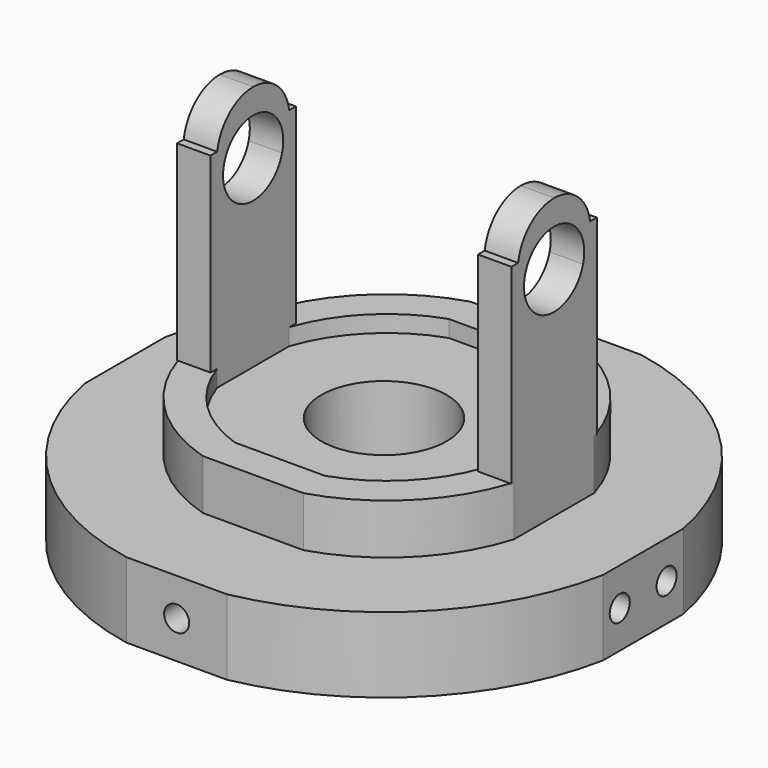
from build123d import *

# Parameters (mm, degrees)
F1_DEPTH  = 6
F2_T      = -4
F3_DEPTH  = 25.4
F4_W      = 10.761987894
F4_H      = 6
F4_H_2    = 27.5
F5_DEPTH  = 4
F6_W      = 10.761987894
F6_H      = 6
F6_H_2    = 27.5
F7_DEPTH  = 4
F9_DEPTH  = 50
F10_DEPTH = 50
F11_DEPTH = 50
F12_DEPTH = 1
F13_DEPTH = 1
F14_DEPTH = 1
F15_DEPTH = 1
F18_DEPTH = 4
F20_DEPTH = 9
F21_R     = 1.5
F22_DEPTH = 7
F23_R     = 1.5
F24_DEPTH = 7
F25_R     = 1.5
F26_DEPTH = 7
F27_R     = 1.5
F28_DEPTH = 7
F29_R     = 7.5
F30_DEPTH = 25.4


with BuildPart() as f1:
    # F0 (on Top) → F1 (new body)
    with BuildSketch(Plane.XY):
        with BuildLine():
            Line((6.0000014261, 20.4372135154), (1.4261e-06, 20.4372135154))
            Line((1.4261e-06, 20.4372135154), (-5.9999985739, 20.4372135154))
            ThreePointArc((-5.9999985739, 20.4372135154), (-14.7648216341, 15.2020365756), (-19.9999985739, 6.4372135154))
            Line((-19.9999985739, 6.4372135154), (-19.9999985739, 0.4372135154))
            Line((-19.9999985739, 0.4372135154), (-19.9999985739, -5.5627864846))
            ThreePointArc((-19.9999985739, -5.5627864846), (-14.7648216341, -14.3276095448), (-5.9999985739, -19.5627864846))
            Line((-5.9999985739, -19.5627864846), (1.4261e-06, -19.5627864846))
            Line((1.4261e-06, -19.5627864846), (6.0000014261, -19.5627864846))
            ThreePointArc((6.0000014261, -19.5627864846), (14.7648244863, -14.3276095448), (20.0000014261, -5.5627864846))
            Line((20.0000014261, -5.5627864846), (20.0000014261, 6.4372135154))
            ThreePointArc((20.0000014261, 6.4372135154), (14.7648244863, 15.2020365756), (6.0000014261, 20.4372135154))
        make_face()
    extrude(amount=F1_DEPTH)

    # F2
    f2_openings = [f1.faces().sort_by_distance(p)[0] for p in [
        (1e-06, 0.437214, 6),
    ]]
    offset(amount=F2_T, openings=f2_openings)

    # F3 (cut): a face of the model
    f3_faces = [f1.faces().sort_by_distance(p)[0] for p in [
        (1.4261e-06, 0.4372135154, 4),
    ]]
    extrude(f3_faces, amount=-F3_DEPTH, mode=Mode.SUBTRACT)

    # F4 (on face) → F5 (join)
    with BuildSketch(Plane(origin=(16.0000014261, 0, 0), x_dir=(0, -1, 0), z_dir=(-1, 0, 0))):
        with Locations((-0.4372135154, 3)):
            Rectangle(F4_W, F4_H)
        with Locations((-0.4372135154, 19.75)):
            Rectangle(F4_W, F4_H_2)
    extrude(amount=-F5_DEPTH)

    # F6 (on face) → F7 (join)
    with BuildSketch(Plane.YZ.offset(-15.9999985739)):
        with Locations((0.4372135154, 3)):
            Rectangle(F6_W, F6_H)
        with Locations((0.4372135154, 19.75)):
            Rectangle(F6_W, F6_H_2)
    extrude(amount=-F7_DEPTH)

    # F8 (on face) → F9 (cut)
    with BuildSketch(Plane(origin=(-19.9999985739, 0, 0), x_dir=(0, -1, 0), z_dir=(-1, 0, 0))):
        with BuildLine():
            Line((-5.8182074624, 33.5), (-5.8182074624, 28.852354537))
            ThreePointArc((-5.8182074624, 28.852354537), (-3.9923402433, 32.177236302), (-0.4372135154, 33.5))
            Line((-0.4372135154, 33.5), (-5.8182074624, 33.5))
        make_face()
    extrude(amount=-F9_DEPTH, mode=Mode.SUBTRACT)

    # F8 (on face) → F10 (cut)
    with BuildSketch(Plane(origin=(-19.9999985739, 0, 0), x_dir=(0, -1, 0), z_dir=(-1, 0, 0))):
        with BuildLine():
            ThreePointArc((-0.4372135154, 33.5), (3.1179132125, 32.177236302), (4.9437804316, 28.852354537))
            Line((4.9437804316, 28.852354537), (4.9437804316, 33.5))
            Line((4.9437804316, 33.5), (-0.4372135154, 33.5))
        make_face()
    extrude(amount=-F10_DEPTH, mode=Mode.SUBTRACT)

    # F8 (on face) → F11 (cut)
    with BuildSketch(Plane(origin=(-19.9999985739, 0, 0), x_dir=(0, -1, 0), z_dir=(-1, 0, 0))):
        with BuildLine():
            ThreePointArc((3.8905718212, 24.7670060502), (4.0195248668, 25.3775186809), (4.0627864846, 26))
            ThreePointArc((4.0627864846, 26), (-1.0596948345, 30.4567383822), (-4.764998852, 24.7670060502))
            ThreePointArc((-4.764998852, 24.7670060502), (-0.4372135154, 21.5), (3.8905718212, 24.7670060502))
        make_face()
    extrude(amount=-F11_DEPTH, mode=Mode.SUBTRACT)

    # F12 (add): a face of the model
    f12_faces = [f1.faces().sort_by_distance(p)[0] for p in [
        (-17.9999985739, 5.8182074624, 17.4261772685),
    ]]
    extrude(f12_faces, amount=F12_DEPTH)

    # F13 (add): a face of the model
    f13_faces = [f1.faces().sort_by_distance(p)[0] for p in [
        (-17.9999985739, -4.9437804316, 17.4261772685),
    ]]
    extrude(f13_faces, amount=F13_DEPTH)

    # F14 (add): a face of the model
    f14_faces = [f1.faces().sort_by_distance(p)[0] for p in [
        (18.0000014261, 5.8182074624, 17.4261772685),
    ]]
    extrude(f14_faces, amount=F14_DEPTH)

    # F15 (add): a face of the model
    f15_faces = [f1.faces().sort_by_distance(p)[0] for p in [
        (18.0000014261, -4.9437804316, 17.4261772685),
    ]]
    extrude(f15_faces, amount=F15_DEPTH)

    # F17 (on face) → F18 (join)
    with BuildSketch(Plane(origin=(0, 0, 0), x_dir=(1, 0, 0), z_dir=(0, 0, -1))):
        with BuildLine():
            Line((1.4261e-06, 15.5627864846), (1.4261e-06, -0.4372135154))
            Line((1.4261e-06, -0.4372135154), (16.0000014261, -0.4372135154))
            Line((16.0000014261, -0.4372135154), (16.0000014261, 4.9437804316))
            ThreePointArc((16.0000014261, 4.9437804316), (11.9363973616, 11.4991824201), (5.3809953731, 15.5627864846))
            Line((5.3809953731, 15.5627864846), (1.4261e-06, 15.5627864846))
        make_face()
        with BuildLine():
            Line((-15.9999985739, 4.9437804316), (-15.9999985739, -0.4372135154))
            Line((-15.9999985739, -0.4372135154), (1.4261e-06, -0.4372135154))
            Line((1.4261e-06, -0.4372135154), (1.4261e-06, 15.5627864846))
            Line((1.4261e-06, 15.5627864846), (-5.3809925209, 15.5627864846))
            ThreePointArc((-5.3809925209, 15.5627864846), (-11.9363945094, 11.4991824201), (-15.9999985739, 4.9437804316))
        make_face()
        with BuildLine():
            Line((1.4261e-06, -0.4372135154), (-15.9999985739, -0.4372135154))
            Line((-15.9999985739, -0.4372135154), (-15.9999985739, -5.8182074624))
            ThreePointArc((-15.9999985739, -5.8182074624), (-11.9363945094, -12.3736094509), (-5.3809925209, -16.4372135154))
            Line((-5.3809925209, -16.4372135154), (1.4261e-06, -16.4372135154))
            Line((1.4261e-06, -16.4372135154), (1.4261e-06, -0.4372135154))
        make_face()
        with BuildLine():
            Line((16.0000014261, -0.4372135154), (1.4261e-06, -0.4372135154))
            Line((1.4261e-06, -0.4372135154), (1.4261e-06, -16.4372135154))
            Line((1.4261e-06, -16.4372135154), (5.3809953731, -16.4372135154))
            ThreePointArc((5.3809953731, -16.4372135154), (11.9363973616, -12.3736094509), (16.0000014261, -5.8182074624))
            Line((16.0000014261, -5.8182074624), (16.0000014261, -0.4372135154))
        make_face()
    extrude(amount=-F18_DEPTH)

    # F19 (on face) → F20 (join)
    with BuildSketch(Plane(origin=(0, 0, 0), x_dir=(1, 0, 0), z_dir=(0, 0, -1))):
        with BuildLine():
            Line((6, 31), (0, 31))
            Line((0, 31), (-6, 31))
            ThreePointArc((-6, 31), (-22.3271135618, 22.3271135618), (-31, 6))
            Line((-31, 6), (-31, -6))
            ThreePointArc((-31, -6), (-22.3271135618, -22.3271135618), (-6, -31))
            Line((-6, -31), (6, -31))
            ThreePointArc((6, -31), (22.3271135618, -22.3271135618), (31, -6))
            Line((31, -6), (31, 0))
            Line((31, 0), (31, 6))
            ThreePointArc((31, 6), (22.3271135618, 22.3271135618), (6, 31))
        make_face()
    extrude(amount=F20_DEPTH)

    # F21 (on face) → F22 (cut)
    with BuildSketch(Plane.XZ.offset(31)):
        with Locations((0, -4.4999574302)):
            Circle(F21_R)
    extrude(amount=-F22_DEPTH, mode=Mode.SUBTRACT)

    # F23 (on face) → F24 (cut)
    with BuildSketch(Plane(origin=(0, 31, 0), x_dir=(-1, 0, 0), z_dir=(0, 1, 0))):
        with Locations((0, -4.5)):
            Circle(F23_R)
    extrude(amount=-F24_DEPTH, mode=Mode.SUBTRACT)

    # F25 (on face) → F26 (cut)
    with BuildSketch(Plane.YZ.offset(31)):
        with Locations((-3.5, -4.5)):
            Circle(F25_R)
        with Locations((3.5, -4.5)):
            Circle(F25_R)
    extrude(amount=-F26_DEPTH, mode=Mode.SUBTRACT)

    # F27 (on face) → F28 (cut)
    with BuildSketch(Plane(origin=(-31, 0, 0), x_dir=(0, -1, 0), z_dir=(-1, 0, 0))):
        with Locations((-3.5, -4.5)):
            Circle(F27_R)
        with Locations((3.5, -4.5)):
            Circle(F27_R)
    extrude(amount=-F28_DEPTH, mode=Mode.SUBTRACT)

    # F29 (on face) → F30 (cut)
    with BuildSketch(Plane.XY.offset(4)):
        Circle(F29_R)
    extrude(amount=-F30_DEPTH, mode=Mode.SUBTRACT)


solid = f1.part
